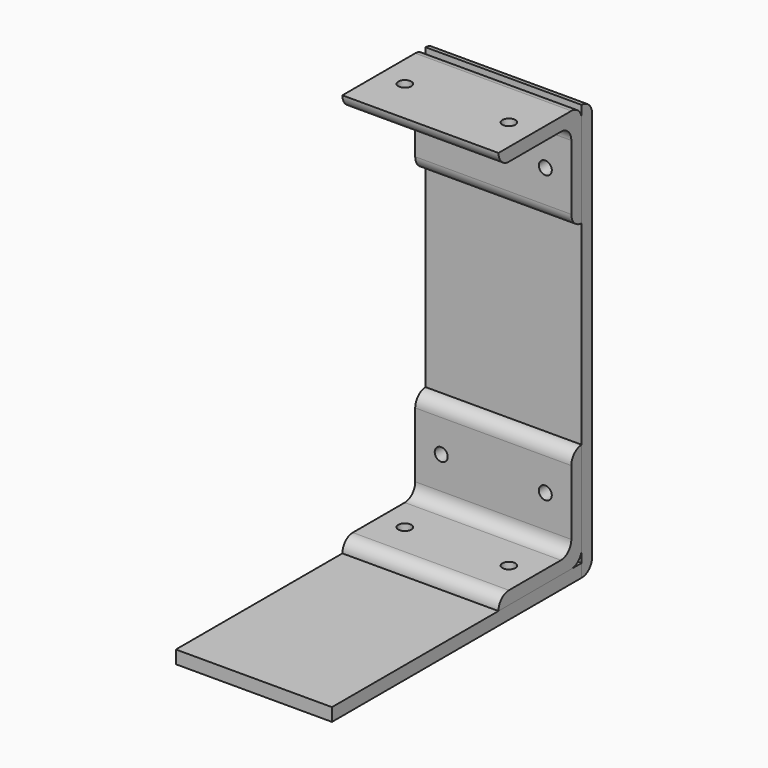
from build123d import *

# Parameters (mm, degrees)
F0_W      = 38.1
F0_H      = 76.2
F1_DEPTH  = 3.175
F3_DEPTH  = 38.1
F4_R      = 1.5875
F5_DEPTH  = 25.4
F6_W      = 38.1
F6_H      = 101.6
F7_DEPTH  = 3.175
F8_R      = 1.5875
F9_DEPTH  = 25.4
F10_R     = 3.17499
F12_DEPTH = 38.1
F13_R     = 1.5875
F15_DEPTH = 25.4
F14_R     = 1.5875
F16_DEPTH = 25.4
F17_R     = 3.17499
F17_2_R   = 3.17499
F18_R     = 3.17499


# Not quite as in the source:
# - a fillet or chamfer is up to 0.001 mm smaller than in the source, because OpenCascade refuses the exact size


with BuildPart() as f1:
    # F0 (on Top) → F1 (new body)
    with BuildSketch(Plane.XY):
        with Locations((2.8697997332, 25.1559876483)):
            Rectangle(F0_W, F0_H)
    extrude(amount=F1_DEPTH)


with BuildPart() as f3:
    # F2 (on face) → F3 (new body)
    with BuildSketch(Plane(origin=(-16.1802002668, 0, 0), x_dir=(0, -1, 0), z_dir=(-1, 0, 0))):
        Polygon((-63.2559876483, 28.575), (-63.2559876483, 3.175), (-37.8559876483, 3.175), (-37.8559876483, 6.35), (-60.0809876483, 6.35), (-60.0809876483, 28.575), align=None)
    extrude(amount=-F3_DEPTH)


with BuildPart() as f5_tool:
    # F4 (on face) → F5 (new body)
    with BuildSketch(Plane.XY.offset(6.35)):
        with Locations((-9.8302002668, 48.9684876483)):
            Circle(F4_R)
        with Locations((15.5697997332, 48.9684876483)):
            Circle(F4_R)
    extrude(amount=-F5_DEPTH)


with BuildPart() as f1_1:
    add(f1.part)

    # F5: cut by f5_tool
    add(f5_tool.part, mode=Mode.SUBTRACT)


with BuildPart() as f3_1:
    add(f3.part)

    # F5: cut by f5_tool
    add(f5_tool.part, mode=Mode.SUBTRACT)


with BuildPart() as f7:
    # F6 (on face) → F7 (new body)
    with BuildSketch(Plane(origin=(0, 63.2559876483, 0), x_dir=(-1, 0, 0), z_dir=(0, 1, 0))):
        with Locations((-2.8697997332, 50.8)):
            Rectangle(F6_W, F6_H)
    extrude(amount=F7_DEPTH)


with BuildPart() as f9_tool:
    # F8 (on face) → F9 (new body)
    with BuildSketch(Plane.XZ.offset(-60.0809876483)):
        with Locations((-9.8302002668, 17.4625)):
            Circle(F8_R)
        with Locations((15.5697997332, 17.4625)):
            Circle(F8_R)
    extrude(amount=-F9_DEPTH)


with BuildPart() as f3_2:
    add(f3_1.part)

    # F9: cut by f9_tool
    add(f9_tool.part, mode=Mode.SUBTRACT)

    # F17#2 (radius 3.175 in the source; OpenCascade refuses exactly that, so slightly less here)
    f17_2_edges = [f3_2.edges().sort_by_distance(p)[0] for p in [
        (2.8698, 60.080988, 28.575),
        (2.8698, 37.855988, 6.35),
        (2.8698, 60.080988, 6.35),
        (2.8698, 63.255988, 3.175),
    ]]
    fillet(f17_2_edges, radius=F17_2_R)


with BuildPart() as f7_1:
    add(f7.part)

    # F9: cut by f9_tool
    add(f9_tool.part, mode=Mode.SUBTRACT)

    # F10 (radius 3.175 in the source; OpenCascade refuses exactly that, so slightly less here)
    f10_edges = [f7_1.edges().sort_by_distance(p)[0] for p in [
        (2.8698, 66.430988, 0),
    ]]
    fillet(f10_edges, radius=F10_R)


with BuildPart() as f12:
    # F11 (on face) → F12 (new body)
    with BuildSketch(Plane.YZ.offset(21.9197997332)):
        Polygon((63.2559876483, 76.2), (63.2559876483, 101.6), (37.8559876483, 101.6), (37.8559876483, 98.425), (60.0809876483, 98.425), (60.0809876483, 76.2), align=None)
    extrude(amount=-F12_DEPTH)


with BuildPart() as f15_tool:
    # F13 (on face) → F15 (new body)
    with BuildSketch(Plane.XZ.offset(-60.0809876483)):
        with Locations((-9.8302002668, 87.3125)):
            Circle(F13_R)
        with Locations((15.5697997332, 87.3125)):
            Circle(F13_R)
    extrude(amount=-F15_DEPTH)


with BuildPart() as f7_2:
    add(f7_1.part)

    # F15: cut by f15_tool
    add(f15_tool.part, mode=Mode.SUBTRACT)

    # F18 (radius 3.175 in the source; OpenCascade refuses exactly that, so slightly less here)
    f18_edges = [f7_2.edges().sort_by_distance(p)[0] for p in [
        (2.8698, 66.430988, 101.6),
    ]]
    fillet(f18_edges, radius=F18_R)


with BuildPart() as f12_1:
    add(f12.part)

    # F15: cut by f15_tool
    add(f15_tool.part, mode=Mode.SUBTRACT)

    # F14 (on face) → F16 (cut)
    with BuildSketch(Plane(origin=(0, 0, 98.425), x_dir=(1, 0, 0), z_dir=(0, 0, -1))):
        with Locations((-9.8302002668, -48.9684876483)):
            Circle(F14_R)
        with Locations((15.5697997332, -48.9684876483)):
            Circle(F14_R)
    extrude(amount=-F16_DEPTH, mode=Mode.SUBTRACT)

    # F17 (radius 3.175 in the source; OpenCascade refuses exactly that, so slightly less here)
    f17_edges = [f12_1.edges().sort_by_distance(p)[0] for p in [
        (2.8698, 60.080988, 98.425),
        (2.8698, 60.080988, 76.2),
        (2.8698, 63.255988, 101.6),
        (2.8698, 37.855988, 98.425),
    ]]
    fillet(f17_edges, radius=F17_R)


solid = Compound([f1_1.part, f3_2.part, f7_2.part, f12_1.part])
